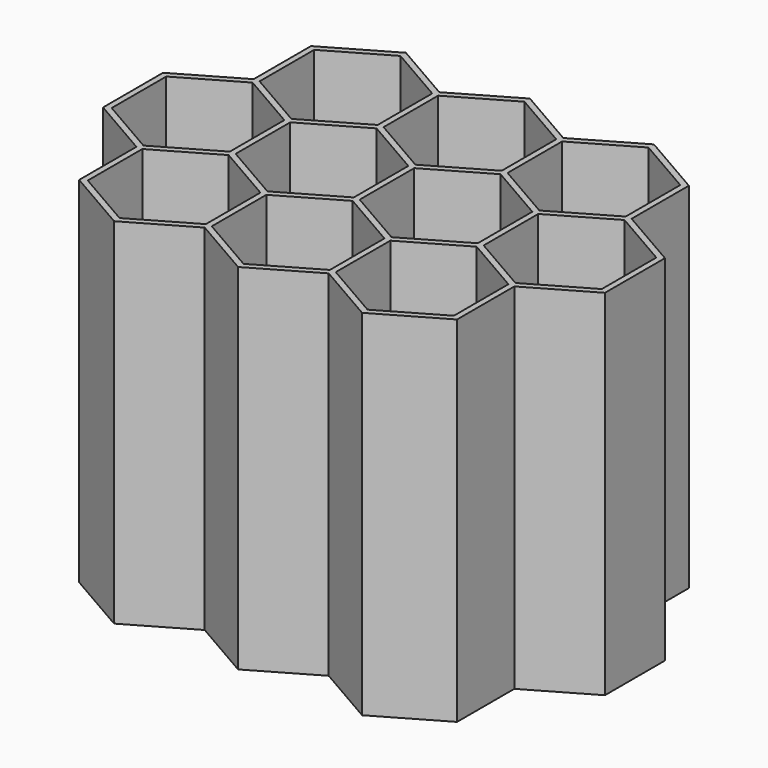
from build123d import *

# Parameters (mm, degrees)
F3_DEPTH = 90
F4_DEPTH = 1.5


with BuildPart() as f3:
    # F1 (on Top) → F3 (new body)
    with BuildSketch(Plane.XY):
        Polygon((0.75, 17.7535207776), (0, 17.3205080757), (15, 8.6602540378), (15, 9.5262794416), (15.75, 9.9592921435), (0.75, 18.6195461814), align=None)
        Polygon((-0.75, 17.7535207776), (0, 17.3205080757), (0.75, 17.7535207776), (0.75, 18.6195461814), (0, 19.0525588833), (-0.75, 18.6195461814), align=None)
        Polygon((-15, 8.6602540378), (0, 17.3205080757), (-0.75, 17.7535207776), (-0.75, 18.6195461814), (-15.75, 9.9592921435), (-16.5, 9.5262794416), (-16.5, 8.6602540378), (-15.75, 8.227241336), align=None)
        Polygon((15.75, 8.227241336), (15, 8.6602540378), (15, -8.6602540378), (15, -9.5262794416), (15.75, -9.9592921435), (16.5, -9.5262794416), (16.5, -8.6602540378), (16.5, 8.6602540378), align=None)
        Polygon((15, 9.5262794416), (15, 8.6602540378), (15.75, 8.227241336), (16.5, 8.6602540378), (16.5, 9.5262794416), (15.75, 9.9592921435), align=None)
        Polygon((-15, -8.6602540378), (-15, 8.6602540378), (-15.75, 8.227241336), (-16.5, 8.6602540378), (-16.5, -9.5262794416), (0, -19.0525588833), (15.75, -9.9592921435), (15, -9.5262794416), (15, -8.6602540378), (0, -17.3205080757), align=None)
        Polygon((0, 19.0525588833), (0.75, 18.6195461814), (0.75, 35.9400542571), (0, 35.5070415552), (-0.75, 35.9400542571), (-0.75, 18.6195461814), align=None)
        Polygon((30.75, 18.6195461814), (15.75, 9.9592921435), (16.5, 9.5262794416), (16.5, 8.6602540378), (31.5, 17.3205080757), (30.75, 17.7535207776), align=None)
        Polygon((-32.25, 17.7535207776), (-16.5, 8.6602540378), (-16.5, 9.5262794416), (-15.75, 9.9592921435), (-30.75, 18.6195461814), (-30.75, 35.9400542571), (-15.75, 44.6003082949), (-16.5, 45.0333209968), (-16.5, 45.8993464006), (-32.25, 36.8060796608), align=None)
        Polygon((0, 35.5070415552), (0.75, 35.9400542571), (0.75, 36.8060796608), (0, 37.2390923627), (-0.75, 36.8060796608), (-0.75, 35.9400542571), align=None)
        Polygon((0.75, 36.8060796608), (0.75, 35.9400542571), (15.75, 44.6003082949), (15, 45.0333209968), (15, 45.8993464006), (0, 37.2390923627), align=None)
        Polygon((-15.75, 44.6003082949), (-0.75, 35.9400542571), (-0.75, 36.8060796608), (0, 37.2390923627), (-15, 45.8993464006), (-15.75, 46.3323591025), (-16.5, 45.8993464006), (-16.5, 45.0333209968), align=None)
        Polygon((16.5, -9.5262794416), (15.75, -9.9592921435), (31.5, -19.0525588833), (47.25, -9.9592921435), (46.5, -9.5262794416), (46.5, -8.6602540378), (31.5, -17.3205080757), (16.5, -8.6602540378), align=None)
        Polygon((30.75, 35.9400542571), (30.75, 18.6195461814), (31.5, 19.0525588833), (32.25, 18.6195461814), (32.25, 35.9400542571), (31.5, 35.5070415552), align=None)
        Polygon((31.5, 19.0525588833), (30.75, 18.6195461814), (30.75, 17.7535207776), (31.5, 17.3205080757), (32.25, 17.7535207776), (32.25, 18.6195461814), align=None)
        Polygon((32.25, 17.7535207776), (31.5, 17.3205080757), (46.5, 8.6602540378), (46.5, 9.5262794416), (47.25, 9.9592921435), (32.25, 18.6195461814), align=None)
        Polygon((16.5, 45.0333209968), (15.75, 44.6003082949), (30.75, 35.9400542571), (30.75, 36.8060796608), (31.5, 37.2390923627), (16.5, 45.8993464006), align=None)
        Polygon((15, 45.0333209968), (15.75, 44.6003082949), (16.5, 45.0333209968), (16.5, 45.8993464006), (15.75, 46.3323591025), (15, 45.8993464006), align=None)
        Polygon((30.75, 36.8060796608), (30.75, 35.9400542571), (31.5, 35.5070415552), (32.25, 35.9400542571), (32.25, 36.8060796608), (31.5, 37.2390923627), align=None)
        Polygon((47.25, 8.227241336), (46.5, 8.6602540378), (46.5, -8.6602540378), (46.5, -9.5262794416), (47.25, -9.9592921435), (48, -9.5262794416), (48, -8.6602540378), (48, 8.6602540378), align=None)
        Polygon((46.5, 9.5262794416), (46.5, 8.6602540378), (47.25, 8.227241336), (48, 8.6602540378), (48, 9.5262794416), (47.25, 9.9592921435), align=None)
        Polygon((48, -9.5262794416), (47.25, -9.9592921435), (63, -19.0525588833), (79.5, -9.5262794416), (79.5, 8.6602540378), (78.75, 8.227241336), (78, 8.6602540378), (78, -8.6602540378), (63, -17.3205080757), (48, -8.6602540378), align=None)
        Polygon((-16.5, 64.08587988), (-16.5, 45.8993464006), (-15.75, 46.3323591025), (-15, 45.8993464006), (-15, 63.2198544763), (0, 71.8801085141), (15, 63.2198544763), (15, 64.08587988), (15.75, 64.5188925819), (0, 73.6121593217), align=None)
        Polygon((15, 63.2198544763), (15, 45.8993464006), (15.75, 46.3323591025), (16.5, 45.8993464006), (16.5, 63.2198544763), (16.5, 64.08587988), (15.75, 64.5188925819), (15, 64.08587988), align=None)
        Polygon((62.25, 18.6195461814), (47.25, 9.9592921435), (48, 9.5262794416), (48, 8.6602540378), (63, 17.3205080757), (62.25, 17.7535207776), align=None)
        Polygon((32.25, 36.8060796608), (32.25, 35.9400542571), (47.25, 44.6003082949), (46.5, 45.0333209968), (46.5, 45.8993464006), (31.5, 37.2390923627), align=None)
        Polygon((16.5, 64.08587988), (16.5, 63.2198544763), (31.5, 71.8801085141), (46.5, 63.2198544763), (46.5, 64.08587988), (47.25, 64.5188925819), (31.5, 73.6121593217), (15.75, 64.5188925819), align=None)
        Polygon((62.25, 35.9400542571), (62.25, 18.6195461814), (63, 19.0525588833), (63.75, 18.6195461814), (63.75, 35.9400542571), (63, 35.5070415552), align=None)
        Polygon((63, 19.0525588833), (62.25, 18.6195461814), (62.25, 17.7535207776), (63, 17.3205080757), (63.75, 17.7535207776), (63.75, 18.6195461814), align=None)
        Polygon((48, 45.0333209968), (47.25, 44.6003082949), (62.25, 35.9400542571), (62.25, 36.8060796608), (63, 37.2390923627), (48, 45.8993464006), align=None)
        Polygon((46.5, 45.0333209968), (47.25, 44.6003082949), (48, 45.0333209968), (48, 45.8993464006), (47.25, 46.3323591025), (46.5, 45.8993464006), align=None)
        Polygon((46.5, 63.2198544763), (46.5, 45.8993464006), (47.25, 46.3323591025), (48, 45.8993464006), (48, 63.2198544763), (48, 64.08587988), (47.25, 64.5188925819), (46.5, 64.08587988), align=None)
        Polygon((63.75, 17.7535207776), (63, 17.3205080757), (78, 8.6602540378), (78.75, 8.227241336), (79.5, 8.6602540378), (79.5, 9.5262794416), (78.75, 9.9592921435), (63.75, 18.6195461814), align=None)
        Polygon((79.5, 9.5262794416), (79.5, 8.6602540378), (95.25, 17.7535207776), (95.25, 36.8060796608), (79.5, 45.8993464006), (79.5, 45.0333209968), (78.75, 44.6003082949), (93.75, 35.9400542571), (93.75, 18.6195461814), (78.75, 9.9592921435), align=None)
        Polygon((62.25, 36.8060796608), (62.25, 35.9400542571), (63, 35.5070415552), (63.75, 35.9400542571), (63.75, 36.8060796608), (63, 37.2390923627), align=None)
        Polygon((63.75, 36.8060796608), (63.75, 35.9400542571), (78.75, 44.6003082949), (79.5, 45.0333209968), (79.5, 45.8993464006), (78.75, 46.3323591025), (78, 45.8993464006), (63, 37.2390923627), align=None)
        Polygon((48, 64.08587988), (48, 63.2198544763), (63, 71.8801085141), (78, 63.2198544763), (78, 45.8993464006), (78.75, 46.3323591025), (79.5, 45.8993464006), (79.5, 64.08587988), (63, 73.6121593217), (47.25, 64.5188925819), align=None)
    extrude(amount=F3_DEPTH)

    # F1 (on Top) → F4 (join)
    with BuildSketch(Plane.XY):
        Polygon((0, 19.0525588833), (0.75, 18.6195461814), (0.75, 35.9400542571), (0, 35.5070415552), (-0.75, 35.9400542571), (-0.75, 18.6195461814), align=None)
        Polygon((30.75, 35.9400542571), (30.75, 18.6195461814), (31.5, 19.0525588833), (32.25, 18.6195461814), (32.25, 35.9400542571), (31.5, 35.5070415552), align=None)
        Polygon((16.5, 63.2198544763), (16.5, 45.8993464006), (31.5, 37.2390923627), (46.5, 45.8993464006), (46.5, 63.2198544763), (31.5, 71.8801085141), align=None)
        Polygon((-15.75, 9.9592921435), (-0.75, 18.6195461814), (-0.75, 35.9400542571), (-15.75, 44.6003082949), (-30.75, 35.9400542571), (-30.75, 18.6195461814), align=None)
        Polygon((-15, 45.8993464006), (0, 37.2390923627), (15, 45.8993464006), (15, 63.2198544763), (0, 71.8801085141), (-15, 63.2198544763), align=None)
        Polygon((15, 8.6602540378), (0, 17.3205080757), (-15, 8.6602540378), (-15, -8.6602540378), (0, -17.3205080757), (15, -8.6602540378), align=None)
        Polygon((63.75, 36.8060796608), (63.75, 35.9400542571), (78.75, 44.6003082949), (79.5, 45.0333209968), (79.5, 45.8993464006), (78.75, 46.3323591025), (78, 45.8993464006), (63, 37.2390923627), align=None)
        Polygon((31.5, 17.3205080757), (16.5, 8.6602540378), (16.5, -8.6602540378), (31.5, -17.3205080757), (46.5, -8.6602540378), (46.5, 8.6602540378), align=None)
        Polygon((63, 17.3205080757), (48, 8.6602540378), (48, -8.6602540378), (63, -17.3205080757), (78, -8.6602540378), (78, 8.6602540378), align=None)
        Polygon((63.75, 35.9400542571), (63.75, 18.6195461814), (78.75, 9.9592921435), (93.75, 18.6195461814), (93.75, 35.9400542571), (78.75, 44.6003082949), align=None)
        Polygon((48, 64.08587988), (48, 63.2198544763), (63, 71.8801085141), (78, 63.2198544763), (78, 45.8993464006), (78.75, 46.3323591025), (79.5, 45.8993464006), (79.5, 64.08587988), (63, 73.6121593217), (47.25, 64.5188925819), align=None)
        Polygon((16.5, 64.08587988), (16.5, 63.2198544763), (31.5, 71.8801085141), (46.5, 63.2198544763), (46.5, 64.08587988), (47.25, 64.5188925819), (31.5, 73.6121593217), (15.75, 64.5188925819), align=None)
        Polygon((-15, -8.6602540378), (-15, 8.6602540378), (-15.75, 8.227241336), (-16.5, 8.6602540378), (-16.5, -9.5262794416), (0, -19.0525588833), (15.75, -9.9592921435), (15, -9.5262794416), (15, -8.6602540378), (0, -17.3205080757), align=None)
        Polygon((-32.25, 17.7535207776), (-16.5, 8.6602540378), (-16.5, 9.5262794416), (-15.75, 9.9592921435), (-30.75, 18.6195461814), (-30.75, 35.9400542571), (-15.75, 44.6003082949), (-16.5, 45.0333209968), (-16.5, 45.8993464006), (-32.25, 36.8060796608), align=None)
        Polygon((16.5, -9.5262794416), (15.75, -9.9592921435), (31.5, -19.0525588833), (47.25, -9.9592921435), (46.5, -9.5262794416), (46.5, -8.6602540378), (31.5, -17.3205080757), (16.5, -8.6602540378), align=None)
        Polygon((48, -9.5262794416), (47.25, -9.9592921435), (63, -19.0525588833), (79.5, -9.5262794416), (79.5, 8.6602540378), (78.75, 8.227241336), (78, 8.6602540378), (78, -8.6602540378), (63, -17.3205080757), (48, -8.6602540378), align=None)
        Polygon((79.5, 9.5262794416), (79.5, 8.6602540378), (95.25, 17.7535207776), (95.25, 36.8060796608), (79.5, 45.8993464006), (79.5, 45.0333209968), (78.75, 44.6003082949), (93.75, 35.9400542571), (93.75, 18.6195461814), (78.75, 9.9592921435), align=None)
        Polygon((-16.5, 64.08587988), (-16.5, 45.8993464006), (-15.75, 46.3323591025), (-15, 45.8993464006), (-15, 63.2198544763), (0, 71.8801085141), (15, 63.2198544763), (15, 64.08587988), (15.75, 64.5188925819), (0, 73.6121593217), align=None)
        Polygon((48, 63.2198544763), (48, 45.8993464006), (63, 37.2390923627), (78, 45.8993464006), (78, 63.2198544763), (63, 71.8801085141), align=None)
        Polygon((0.75, 35.9400542571), (0.75, 18.6195461814), (15.75, 9.9592921435), (30.75, 18.6195461814), (30.75, 35.9400542571), (15.75, 44.6003082949), align=None)
        Polygon((32.25, 35.9400542571), (32.25, 18.6195461814), (47.25, 9.9592921435), (62.25, 18.6195461814), (62.25, 35.9400542571), (47.25, 44.6003082949), align=None)
        Polygon((46.5, 45.0333209968), (47.25, 44.6003082949), (48, 45.0333209968), (48, 45.8993464006), (47.25, 46.3323591025), (46.5, 45.8993464006), align=None)
        Polygon((15, 45.0333209968), (15.75, 44.6003082949), (16.5, 45.0333209968), (16.5, 45.8993464006), (15.75, 46.3323591025), (15, 45.8993464006), align=None)
        Polygon((62.25, 36.8060796608), (62.25, 35.9400542571), (63, 35.5070415552), (63.75, 35.9400542571), (63.75, 36.8060796608), (63, 37.2390923627), align=None)
        Polygon((-0.75, 17.7535207776), (0, 17.3205080757), (0.75, 17.7535207776), (0.75, 18.6195461814), (0, 19.0525588833), (-0.75, 18.6195461814), align=None)
        Polygon((15, 9.5262794416), (15, 8.6602540378), (15.75, 8.227241336), (16.5, 8.6602540378), (16.5, 9.5262794416), (15.75, 9.9592921435), align=None)
        Polygon((31.5, 19.0525588833), (30.75, 18.6195461814), (30.75, 17.7535207776), (31.5, 17.3205080757), (32.25, 17.7535207776), (32.25, 18.6195461814), align=None)
        Polygon((46.5, 9.5262794416), (46.5, 8.6602540378), (47.25, 8.227241336), (48, 8.6602540378), (48, 9.5262794416), (47.25, 9.9592921435), align=None)
        Polygon((63, 19.0525588833), (62.25, 18.6195461814), (62.25, 17.7535207776), (63, 17.3205080757), (63.75, 17.7535207776), (63.75, 18.6195461814), align=None)
        Polygon((0, 35.5070415552), (0.75, 35.9400542571), (0.75, 36.8060796608), (0, 37.2390923627), (-0.75, 36.8060796608), (-0.75, 35.9400542571), align=None)
        Polygon((30.75, 36.8060796608), (30.75, 35.9400542571), (31.5, 35.5070415552), (32.25, 35.9400542571), (32.25, 36.8060796608), (31.5, 37.2390923627), align=None)
    extrude(amount=F4_DEPTH)


solid = f3.part
